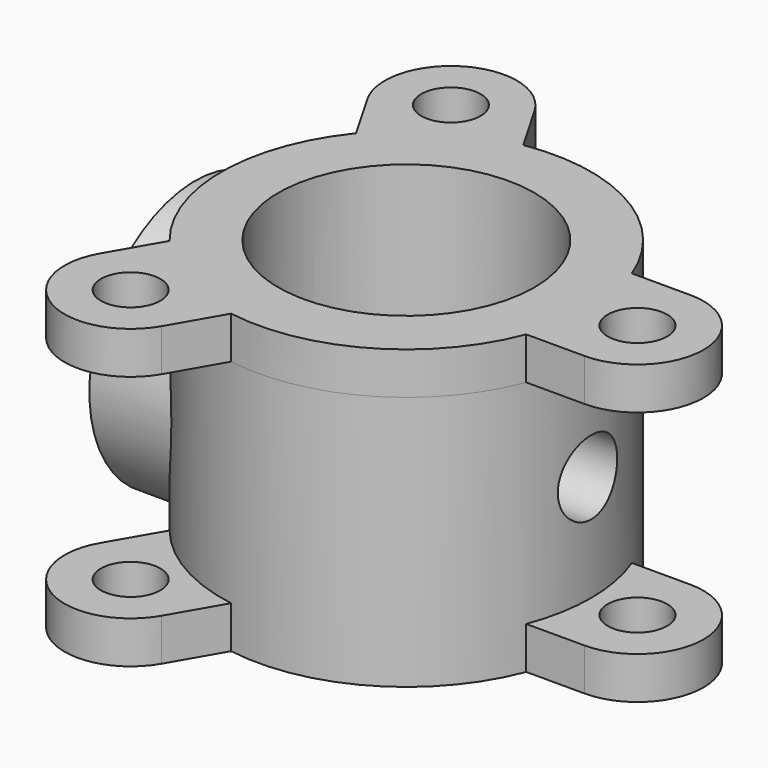
from build123d import *

# Parameters (mm, degrees)
F0_R            = 140
F0_R_2          = 97
F1_DEPTH        = 112.5
F2_R            = 22.5
F3_DEPTH        = 32
F3_COPIES_COUNT = 3
F5_R            = 100
F7_R            = 28.1
F8_DEPTH        = 310
F9_R            = 50
F9_R_2          = 28.1
F10_DEPTH       = 25
F11_R           = 10.15
F12_DEPTH       = 15
F14_R           = 22.5
F14_R_2         = 97
F15_DEPTH       = 32


# Not quite as in the source:
# - a pattern or mirror of a feature is missing from the dataset's text; its kind, count and spacing are read off the source's solid
# - a feature names something its author has since deleted; it is built from what else it names


with BuildPart() as f1:
    # F0 (on Top) → F1 (new body, symmetric)
    with BuildSketch(Plane.XY):
        Circle(F0_R)
        Circle(F0_R_2, mode=Mode.SUBTRACT)
    extrude(amount=F1_DEPTH, both=True)

    # F2 (on face) → F3 (join)
    with BuildSketch(Plane(origin=(0, 0, -112.5), x_dir=(1, 0, 0), z_dir=(0, 0, -1))):
        with BuildLine():
            ThreePointArc((-44.1987298108, 176.5544456623), (-112.5, 194.8557158515), (-130.8012701892, 126.5544456623))
            Line((-130.8012701892, 126.5544456623), (-108.6847543423, 88.2475165291))
            ThreePointArc((-108.6847543423, 88.2475165291), (-70, 121.2435565298), (-22.0822139639, 138.2475165291))
            Line((-22.0822139639, 138.2475165291), (-44.1987298108, 176.5544456623))
        make_face()
        with Locations((-87.5, 151.5544456623)):
            Circle(F2_R, mode=Mode.SUBTRACT)
    f3 = extrude(amount=-F3_DEPTH)

    # F3_copies: F3 ×3 about axis
    f3_copies_axis = Axis((0, 0, 0), (0, 0, 1))
    for i in range(1, F3_COPIES_COUNT):
        add(f3.rotate(f3_copies_axis, i * 360 / F3_COPIES_COUNT))

    # F5 (on offset) → F6 (join, up to the next surface of F1)
    with BuildSketch(Plane.YZ.offset(-160)):
        Circle(F5_R)
    extrude(until=Until.NEXT)

    # F7 (on face) → F8 (cut)
    with BuildSketch(Plane(origin=(-160, 0, 0), x_dir=(0, -1, 0), z_dir=(-1, 0, 0))):
        Circle(F7_R)
    extrude(amount=-F8_DEPTH, mode=Mode.SUBTRACT)

    # F9 (on face) → F10 (cut)
    with BuildSketch(Plane(origin=(-160, 0, 0), x_dir=(0, -1, 0), z_dir=(-1, 0, 0))):
        Circle(F9_R)
        Circle(F9_R_2, mode=Mode.SUBTRACT)
    extrude(amount=-F10_DEPTH, mode=Mode.SUBTRACT)

    # F11 (on face) → F12 (cut)
    with BuildSketch(Plane(origin=(-160, 0, 0), x_dir=(0, -1, 0), z_dir=(-1, 0, 0))):
        with Locations((0, 79.0973976254)):
            Circle(F11_R)
        with Locations((-68.5003557169, -39.5486988127)):
            Circle(F11_R)
        with Locations((68.5003557169, -39.5486988127)):
            Circle(F11_R)
    extrude(amount=-F12_DEPTH, mode=Mode.SUBTRACT)

    # F14 (on face) → F15 (join)
    with BuildSketch(Plane.XY.offset(112.5)):
        with BuildLine():
            Line((-130.8012701892, 126.5544456623), (-108.6847543423, 88.2475165291))
            ThreePointArc((-108.6847543423, 88.2475165291), (-70, 121.2435565298), (-22.0822139639, 138.2475165291))
            Line((-22.0822139639, 138.2475165291), (-44.1987298108, 176.5544456623))
            ThreePointArc((-44.1987298108, 176.5544456623), (-112.5, 194.8557158515), (-130.8012701892, 126.5544456623))
        make_face()
        with Locations((-87.5, 151.5544456623)):
            Circle(F14_R, mode=Mode.SUBTRACT)
        with BuildLine():
            ThreePointArc((-22.0822139639, 138.2475165291), (-70, 121.2435565298), (-108.6847543423, 88.2475165291))
            ThreePointArc((-108.6847543423, 88.2475165291), (-140, 0), (-108.6847543423, -88.2475165291))
            ThreePointArc((-108.6847543423, -88.2475165291), (-70, -121.2435565298), (-22.0822139639, -138.2475165291))
            ThreePointArc((-22.0822139639, -138.2475165291), (70, -121.2435565298), (130.7669683062, -50))
            ThreePointArc((130.7669683062, -50), (137.6723929531, -25.4226713499), (140, 0))
            ThreePointArc((140, 0), (137.6723929531, 25.4226713499), (130.7669683062, 50))
            ThreePointArc((130.7669683062, 50), (70, 121.2435565298), (-22.0822139639, 138.2475165291))
        make_face()
        Circle(F14_R_2, mode=Mode.SUBTRACT)
        with BuildLine():
            ThreePointArc((-22.0822139639, -138.2475165291), (-70, -121.2435565298), (-108.6847543423, -88.2475165291))
            Line((-108.6847543423, -88.2475165291), (-130.8012701892, -126.5544456623))
            ThreePointArc((-130.8012701892, -126.5544456623), (-112.5, -194.8557158515), (-44.1987298108, -176.5544456623))
            Line((-44.1987298108, -176.5544456623), (-22.0822139639, -138.2475165291))
        make_face()
        with Locations((-87.5, -151.5544456623)):
            Circle(F14_R, mode=Mode.SUBTRACT)
        with BuildLine():
            Line((175, 50), (130.7669683062, 50))
            ThreePointArc((130.7669683062, 50), (137.6723929531, 25.4226713499), (140, 0))
            ThreePointArc((140, 0), (137.6723929531, -25.4226713499), (130.7669683062, -50))
            Line((130.7669683062, -50), (175, -50))
            ThreePointArc((175, -50), (225, 0), (175, 50))
        make_face()
        with Locations((175, 0)):
            Circle(F14_R, mode=Mode.SUBTRACT)
    extrude(amount=-F15_DEPTH)


solid = f1.part
